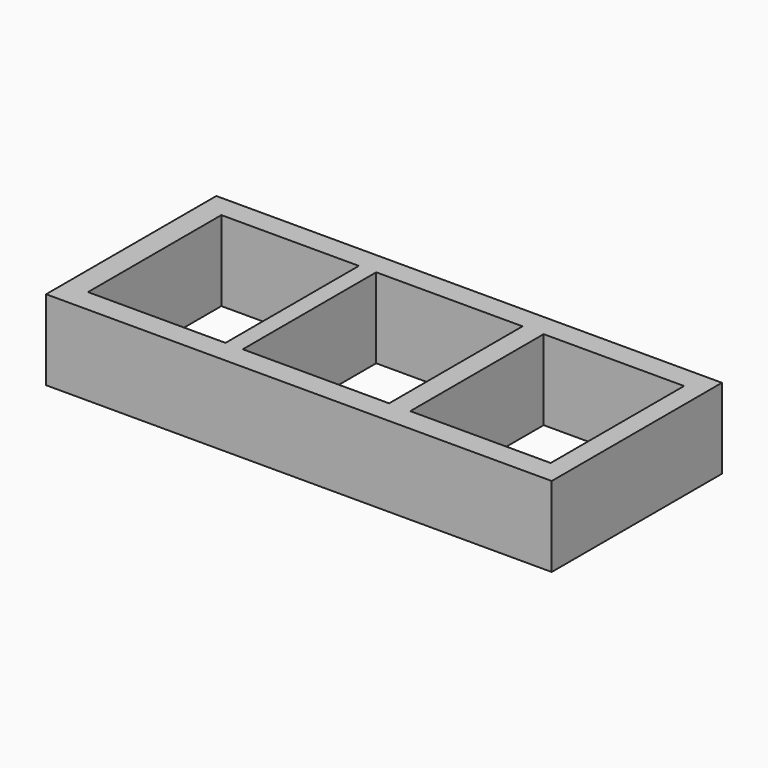
from build123d import *

# Parameters (mm, degrees)
F0_W     = 11861.8
F0_H     = 4991.1
F0_W_2   = 3225.8
F0_H_2   = 3911.6
F0_W_3   = 3432.8365325928
F0_W_4   = 3293.9357757568
F1_DEPTH = 1879.6


# Not quite as in the source:
# - the program builds the solid bodies; features that only make, move or delete a surface that nothing else refers to are left out


with BuildPart() as f1:
    # F0 (on Top) → F1 (new body)
    with BuildSketch(Plane.XY):
        with Locations((3599.2848639578, 1395.0591189232)):
            Rectangle(F0_W, F0_H)
        with Locations((-172.6151360422, 1401.4091189232)):
            Rectangle(F0_W_2, F0_H_2, mode=Mode.SUBTRACT)
        with Locations((3562.8583431244, 1401.4091189232)):
            Rectangle(F0_W_3, F0_H_2, mode=Mode.SUBTRACT)
        with Locations((7422.3194122314, 1401.4091189232)):
            Rectangle(F0_W_4, F0_H_2, mode=Mode.SUBTRACT)
    extrude(amount=F1_DEPTH)


solid = f1.part
